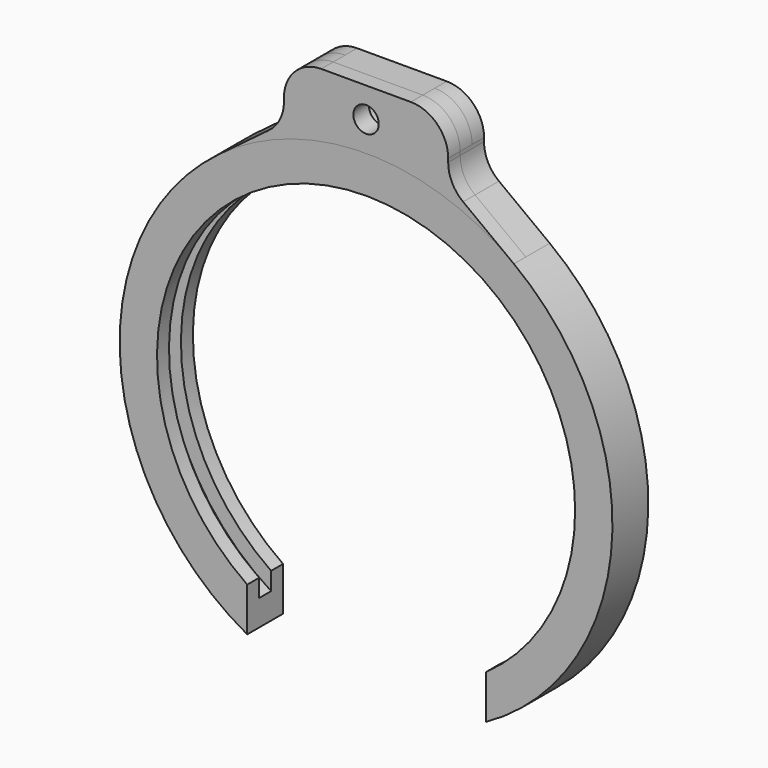
from build123d import *

# Parameters (mm, degrees)
F0_R            = 28
F1_DEPTH        = 2
F2_R            = 30
F2_R_2          = 1.5
F3_DEPTH        = 2
F4_R            = 30
F4_R_2          = 28
F5_DEPTH        = 2
F6_DEPTH        = 2
F7_T1_DEPTH     = 14.5
F7_T3_DEPTH     = 2
F7_T5_DEPTH     = 14.5
F8_T1_DEPTH     = 14.5
F8_T3_DEPTH     = 2
F8_T5_DEPTH     = 14.5
F10_DEPTH       = 6
F11_D           = 3.4
F11_CBORE_D     = 6.4
F11_CBORE_DEPTH = 3.4


# Not quite as in the source:
# - a fillet or chamfer that OpenCascade refuses, or shapes differently, is made with other operations: its cross-section is extruded or revolved along the edge and cut away or added


with BuildPart() as f1:
    # F0 (on Front) → F1 (new body)
    with BuildSketch(Plane.XZ):
        with BuildLine():
            ThreePointArc((-19.8, 26.4), (-14.7580486515, -29.516097303), (33, 0))
            ThreePointArc((33, 0), (29.516097303, 14.7580486515), (19.8, 26.4))
            ThreePointArc((19.8, 26.4), (10.4355162786, 31.3065488357), (0, 33))
            ThreePointArc((0, 33), (-10.4355162786, 31.3065488357), (-19.8, 26.4))
        make_face()
        Circle(F0_R, mode=Mode.SUBTRACT)
        with BuildLine():
            Line((-13, 31.5), (-19.8, 26.4))
            ThreePointArc((-19.8, 26.4), (-10.4355162786, 31.3065488357), (0, 33))
            Line((0, 33), (0, 35.5))
            ThreePointArc((0, 35.5), (-1.5, 37), (0, 38.5))
            Line((0, 38.5), (0, 41))
            Line((0, 41), (-11, 41))
            Line((-11, 41), (-11, 35.5))
            ThreePointArc((-11, 35.5), (-11.527864045, 33.2639320225), (-13, 31.5))
        make_face()
        with BuildLine():
            ThreePointArc((0, 33), (10.4355162786, 31.3065488357), (19.8, 26.4))
            Line((19.8, 26.4), (13, 31.5))
            ThreePointArc((13, 31.5), (11.527864045, 33.2639320225), (11, 35.5))
            Line((11, 35.5), (11, 41))
            Line((11, 41), (0, 41))
            Line((0, 41), (0, 38.5))
            ThreePointArc((0, 38.5), (1.0606601718, 38.0606601718), (1.5, 37))
            ThreePointArc((1.5, 37), (1.0606601718, 35.9393398282), (0, 35.5))
            Line((0, 35.5), (0, 33))
        make_face()
    extrude(amount=F1_DEPTH)

    # F2 (on face) → F3 (join)
    with BuildSketch(Plane.XZ.offset(2)):
        with BuildLine():
            Line((11, 41), (-11, 41))
            Line((-11, 41), (-11, 35.5))
            ThreePointArc((-11, 35.5), (-11.527864045, 33.2639320225), (-13, 31.5))
            Line((-13, 31.5), (-19.8, 26.4))
            ThreePointArc((-19.8, 26.4), (0, -33), (19.8, 26.4))
            Line((19.8, 26.4), (13, 31.5))
            ThreePointArc((13, 31.5), (11.527864045, 33.2639320225), (11, 35.5))
            Line((11, 35.5), (11, 41))
        make_face()
        Circle(F2_R, mode=Mode.SUBTRACT)
        with Locations((0, 37)):
            Circle(F2_R_2, mode=Mode.SUBTRACT)
    extrude(amount=F3_DEPTH)

    # F4 (on face) → F5 (join)
    with BuildSketch(Plane.XZ.offset(4)):
        with BuildLine():
            ThreePointArc((-19.8, 26.4), (-14.7580486515, -29.516097303), (33, 0))
            ThreePointArc((33, 0), (29.516097303, 14.7580486515), (19.8, 26.4))
            ThreePointArc((19.8, 26.4), (0, 33), (-19.8, 26.4))
        make_face()
        Circle(F4_R, mode=Mode.SUBTRACT)
        Circle(F4_R)
        Circle(F4_R_2, mode=Mode.SUBTRACT)
    extrude(amount=F5_DEPTH)

    # F6 (add): a face of the model
    f6_faces = [f1.faces().sort_by_distance(p)[0] for p in [
        (10.5779431318, -4, 38.25),
    ]]
    extrude(f6_faces, amount=F6_DEPTH)

    # F7: fillet of radius 5 on 3 edges, made by hand

    # F7_s2 → F7_t1 (cut)
    with BuildSketch(Plane.XZ.offset(-12.5)):
        with BuildLine():
            ThreePointArc((-11, 36), (-9.5355339059, 39.5355339059), (-6, 41))
            Line((-6, 41), (-11, 41))
            Line((-11, 41), (-11, 36))
        make_face()
    extrude(amount=F7_T1_DEPTH, mode=Mode.SUBTRACT)

    # F7_s4 → F7_t3 (cut)
    with BuildSketch(Plane.XZ.offset(2)):
        with BuildLine():
            ThreePointArc((-11, 36), (-9.5355339059, 39.5355339059), (-6, 41))
            Line((-6, 41), (-11, 41))
            Line((-11, 41), (-11, 36))
        make_face()
    extrude(amount=F7_T3_DEPTH, mode=Mode.SUBTRACT)

    # F7_s6 → F7_t5 (cut)
    with BuildSketch(Plane.XZ.offset(4)):
        with BuildLine():
            ThreePointArc((-11, 36), (-9.5355339059, 39.5355339059), (-6, 41))
            Line((-6, 41), (-11, 41))
            Line((-11, 41), (-11, 36))
        make_face()
    extrude(amount=F7_T5_DEPTH, mode=Mode.SUBTRACT)

    # F8: fillet of radius 5 on 3 edges, made by hand

    # F8_s2 → F8_t1 (cut)
    with BuildSketch(Plane.XZ.offset(-12.5)):
        with BuildLine():
            ThreePointArc((6, 41), (9.5355339059, 39.5355339059), (11, 36))
            Line((11, 36), (11, 41))
            Line((11, 41), (6, 41))
        make_face()
    extrude(amount=F8_T1_DEPTH, mode=Mode.SUBTRACT)

    # F8_s4 → F8_t3 (cut)
    with BuildSketch(Plane.XZ.offset(2)):
        with BuildLine():
            ThreePointArc((6, 41), (9.5355339059, 39.5355339059), (11, 36))
            Line((11, 36), (11, 41))
            Line((11, 41), (6, 41))
        make_face()
    extrude(amount=F8_T3_DEPTH, mode=Mode.SUBTRACT)

    # F8_s6 → F8_t5 (cut)
    with BuildSketch(Plane.XZ.offset(4)):
        with BuildLine():
            ThreePointArc((6, 41), (9.5355339059, 39.5355339059), (11, 36))
            Line((11, 36), (11, 41))
            Line((11, 41), (6, 41))
        make_face()
    extrude(amount=F8_T5_DEPTH, mode=Mode.SUBTRACT)

    # F9 (on face) → F10 (cut)
    with BuildSketch(Plane.XZ.offset(6)):
        with BuildLine():
            ThreePointArc((16.0808527693, -22.9217402091), (0.0985229196, -27.9998266644), (-15.9191472307, -23.0343385285))
            Line((-15.9191472307, -23.0343385285), (-15.9191472307, -28.9064136732))
            ThreePointArc((-15.9191472307, -28.9064136732), (0.0924457314, -32.9998705117), (16.0808527693, -28.8167689759))
            Line((16.0808527693, -28.8167689759), (16.0808527693, -22.9217402091))
        make_face()
    extrude(amount=-F10_DEPTH, mode=Mode.SUBTRACT)

    # F11 (through all)
    with Locations(Plane(origin=(0, 0, 0), x_dir=(1, 0, 0), z_dir=(0, 1, 0))):
        with Locations((0, -37)):
            CounterBoreHole(F11_D / 2, F11_CBORE_D / 2, F11_CBORE_DEPTH)


solid = f1.part
